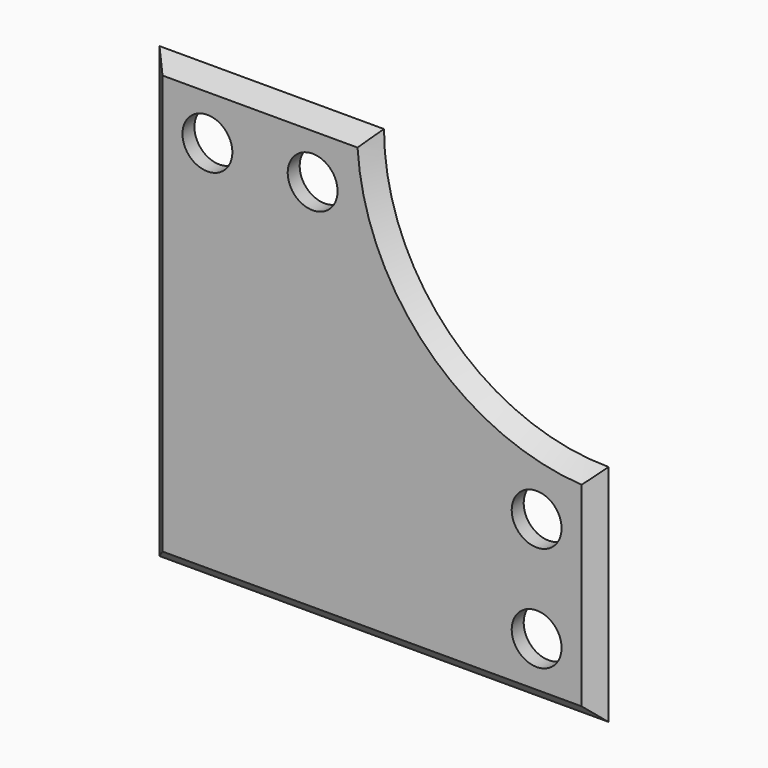
from build123d import *

# Parameters (mm, degrees)
F1_DEPTH = 3
F2_SIZE  = 2.99999
F4_D     = 10
F4_DEPTH = 9
F4_TIP   = 3.0043030951


# Not quite as in the source:
# - a fillet or chamfer is up to 0.001 mm smaller than in the source, because OpenCascade refuses the exact size


with BuildPart() as f1:
    # F0 (on Front) → F1 (new body)
    with BuildSketch(Plane.XZ):
        with BuildLine():
            Line((0, 90), (0, 0))
            Line((0, 0), (90, 0))
            Line((90, 0), (90, 45))
            ThreePointArc((90, 45), (58.1801948466, 58.1801948466), (45, 90))
            Line((45, 90), (0, 90))
        make_face()
    extrude(amount=F1_DEPTH)

    # F2 (size 3 in the source; OpenCascade refuses exactly that, so slightly less here)
    f2_edges = [f1.edges().sort_by_distance(p)[0] for p in [
        (22.5, -3, 90),
        (0, -3, 45),
        (45, -3, 0),
        (90, -3, 22.5),
        (58.180195, -3, 58.180195),
    ]]
    chamfer(f2_edges, length=F2_SIZE)

    # F4
    with Locations(Plane.XZ.offset(3)):
        with Locations((12, 78), (33.093841732, 78), (78, 33.093841732), (78, 12)):
            Hole(F4_D / 2, depth=F4_DEPTH)
            with Locations((0, 0, -(F4_DEPTH + F4_TIP / 2))):  # 118° drill point
                Cone(0, F4_D / 2, F4_TIP, mode=Mode.SUBTRACT)


solid = f1.part
